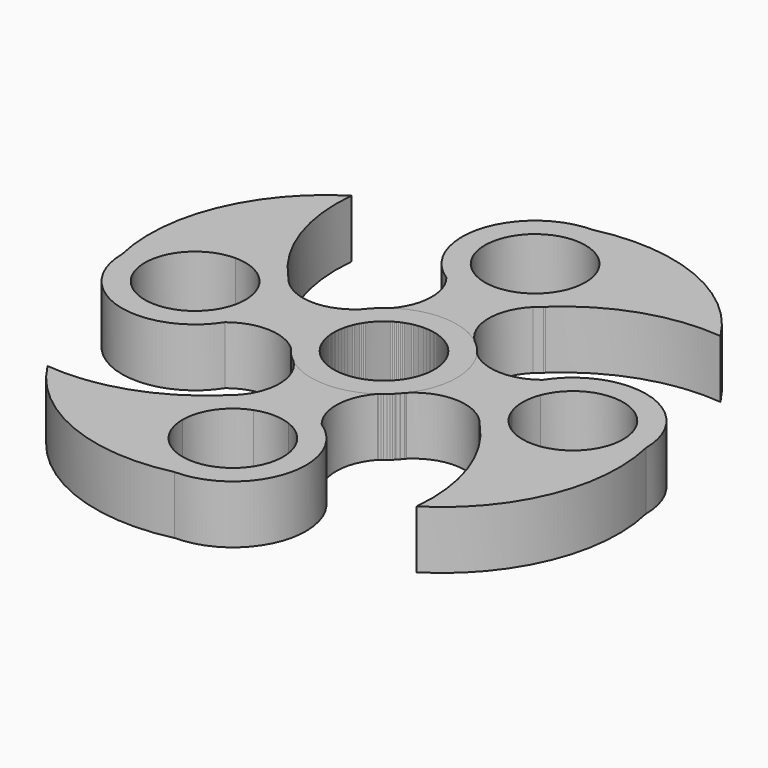
from build123d import *

# Parameters (mm, degrees)
F0_R     = 10.9982
F1_DEPTH = 12.7
F3_COUNT = 4


# Not quite as in the source:
# - a length typed as a fraction of an inch, garbled in the dataset ("3 / 203.2 mm" for 3/8 in), is restored


with BuildPart() as f1:
    # F0 (on Top) → F1 (new body)
    with BuildSketch(Plane.XY):
        with BuildLine():
            ThreePointArc((-9.0574669333, 13.0830533178), (-7.3850555796, -14.0948552831), (15.9123848422, 0))
            ThreePointArc((15.9123848422, 0), (14.6460054276, 6.2208131607), (11.0484355643, 11.451465537))
            ThreePointArc((11.0484355643, 11.451465537), (10.3434763018, 12.0113676326), (9.6851617696, 12.6254359474))
            ThreePointArc((9.6851617696, 12.6254359474), (0.3883987851, 15.9076440037), (-9.0574669333, 13.0830533178))
        make_face()
        Circle(F0_R, mode=Mode.SUBTRACT)
        with BuildLine():
            ThreePointArc((9.6851617696, 12.6254359474), (10.3434763018, 12.0113676326), (11.0484355643, 11.451465537))
            ThreePointArc((11.0484355643, 11.451465537), (10.3834034032, 12.0577330014), (9.6851617696, 12.6254359474))
        make_face()
        with BuildLine():
            ThreePointArc((-8.6296886983, 27.851621109), (-6.1388654172, 20.3889939974), (-9.0574669333, 13.0830533178))
            ThreePointArc((-9.0574669333, 13.0830533178), (0.3883987851, 15.9076440037), (9.6851617696, 12.6254359474))
            ThreePointArc((9.6851617696, 12.6254359474), (6.4040035107, 20.6317448662), (9.7260774595, 28.621163287))
            ThreePointArc((9.7260774595, 28.621163287), (0.6697506027, 25.3369311259), (-8.6296886983, 27.851621109))
        make_face()
        with BuildLine():
            ThreePointArc((0, 57.3018716166), (-15.3442886931, 45.8086601687), (-8.6296886983, 27.851621109))
            ThreePointArc((-8.6296886983, 27.851621109), (0.6697506027, 25.3369311259), (9.7260774595, 28.621163287))
            ThreePointArc((9.7260774595, 28.621163287), (10.3654764315, 29.2130158448), (11.0484355643, 29.7540216843))
            ThreePointArc((11.0484355643, 29.7540216843), (14.7024232976, 35.0272884636), (15.9894867744, 41.3123848422))
            ThreePointArc((15.9894867744, 41.3123848422), (11.3062745259, 52.6186593681), (0, 57.3018716166))
        make_face()
        with BuildLine():
            ThreePointArc((-3.9496509434, 31.0478507239), (-6.2258072663, 50.3787913587), (10.9982, 41.3123848422))
            ThreePointArc((10.9982, 41.3123848422), (9.0089722253, 35.0037540332), (3.7608661302, 30.9771882214))
            ThreePointArc((3.7608661302, 30.9771882214), (-0.1008207719, 30.3110721933), (-3.9496509434, 31.0478507239))
        make_face(mode=Mode.SUBTRACT)
        with BuildLine():
            ThreePointArc((11.0484355643, 29.7540216843), (10.3654764315, 29.2130158448), (9.7260774595, 28.621163287))
            ThreePointArc((9.7260774595, 28.621163287), (10.4026890697, 29.1695784356), (11.0484355643, 29.7540216843))
        make_face()
        with BuildLine():
            ThreePointArc((11.3013842763, 29.9936286052), (14.9309817334, 47.4883530697), (0, 57.3018716166))
            ThreePointArc((0, 57.3018716166), (11.3062745259, 52.6186593681), (15.9894867744, 41.3123848422))
            ThreePointArc((15.9894867744, 41.3123848422), (14.7024232976, 35.0272884636), (11.0484355643, 29.7540216843))
            ThreePointArc((11.0484355643, 29.7540216843), (11.1746387033, 29.8741114636), (11.3013842763, 29.9936286052))
        make_face()
        with BuildLine():
            ThreePointArc((41.404497074, 40.231774447), (23.4329572677, 55.3903132514), (0, 57.3018716166))
            ThreePointArc((0, 57.3018716166), (14.9309817334, 47.4883530697), (11.3013842763, 29.9936286052))
            ThreePointArc((11.3013842763, 29.9936286052), (25.2458915004, 38.367746599), (41.404497074, 40.231774447))
        make_face()
        with BuildLine():
            ThreePointArc((11.3013842763, 29.9936286052), (11.1746387033, 29.8741114636), (11.0484355643, 29.7540216843))
            ThreePointArc((11.0484355643, 29.7540216843), (11.175566557, 29.8731319451), (11.3013842763, 29.9936286052))
        make_face()
    extrude(amount=F1_DEPTH)


with BuildPart() as f3_1:
    # F3: instance of F1
    add(f1.part.rotate(Axis((0, 0, -12.2091118246), (0, 0, -1)), 1 * 360 / F3_COUNT))


with BuildPart() as f3_2:
    # F3: instance of F1
    add(f1.part.rotate(Axis((0, 0, -12.2091118246), (0, 0, -1)), 2 * 360 / F3_COUNT))


with BuildPart() as f3_3:
    # F3: instance of F1
    add(f1.part.rotate(Axis((0, 0, -12.2091118246), (0, 0, -1)), 3 * 360 / F3_COUNT))


solid = Compound([f1.part, f3_1.part, f3_2.part, f3_3.part])
